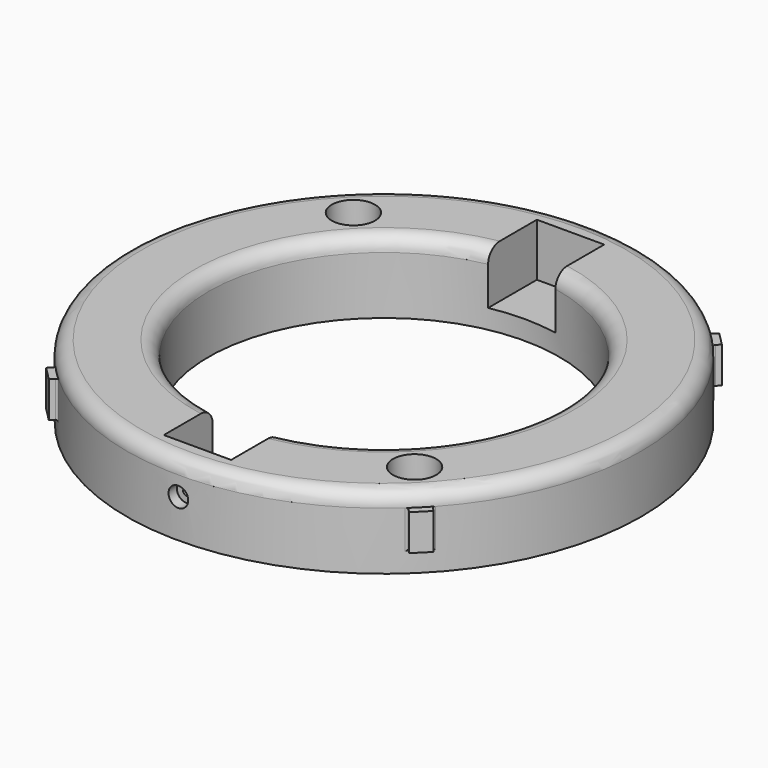
from build123d import *

# Parameters (mm, degrees)
F0_R             = 53.5
F0_R_2           = 36.5
F1_DEPTH         = 15
F5_D             = 6
F5_CBORE_D       = 9
F5_CBORE_DEPTH   = 5
F7_W             = 14
F7_H             = 11
F8_DEPTH         = 15
F10_W            = 14
F10_H            = 11
F11_DEPTH        = 15
F13_R            = 2.05
F14_DEPTH        = 2.2
F16_R            = 2.05
F17_DEPTH        = 2.2
F18_R            = 3
F19_DEPTH        = 7.5
F20_DEPTH        = 7.5
F21_R            = 3
F22_R            = 3
F25_W            = 4
F25_H            = 7.5
F26_DEPTH        = 1.5
F26_COPIES_COUNT = 4
F27_R            = 0.5
F29_D            = 1.5


# Not quite as in the source:
# - a pattern or mirror of a feature is missing from the dataset's text; its kind, count and spacing are read off the source's solid


with BuildPart() as f1:
    # F0 (on Top) → F1 (new body)
    with BuildSketch(Plane.XY):
        Circle(F0_R)
        Circle(F0_R_2, mode=Mode.SUBTRACT)
    extrude(amount=F1_DEPTH)

    # F5 (through all)
    with Locations(Plane.XY.offset(15)):
        with Locations((-31.8198051534, 31.8198051534), (31.8198051534, -31.8198051534)):
            CounterBoreHole(F5_D / 2, F5_CBORE_D / 2, F5_CBORE_DEPTH)

    # F7 (on plane+point) → F8 (cut)
    with BuildSketch(Plane.XZ.offset(-33.5)):
        with Locations((0, 9.5)):
            Rectangle(F7_W, F7_H)
    extrude(amount=-F8_DEPTH, mode=Mode.SUBTRACT)

    # F10 (on plane+point) → F11 (cut)
    with BuildSketch(Plane.XZ.offset(33.5)):
        with Locations((0, 9.5)):
            Rectangle(F10_W, F10_H)
    extrude(amount=F11_DEPTH, mode=Mode.SUBTRACT)

    # F13 (on plane+point) → F14 (cut)
    with BuildSketch(Plane.XZ.offset(53.5)):
        with Locations((0, 8)):
            Circle(F13_R)
    extrude(amount=-F14_DEPTH, mode=Mode.SUBTRACT)

    # F16 (on plane+point) → F17 (cut)
    with BuildSketch(Plane.XZ.offset(-53.5)):
        with Locations((0, 8)):
            Circle(F16_R)
    extrude(amount=F17_DEPTH, mode=Mode.SUBTRACT)

    # F18 (on face) → F19 (cut)
    with BuildSketch(Plane(origin=(0, 0, 0), x_dir=(1, 0, 0), z_dir=(0, 0, -1))):
        Polygon((-33.2340187158, -24.0416305603), (-39.5979797464, -30.405591591), (-30.405591591, -39.5979797464), (-24.0416305603, -33.2340187158), align=None)
        with Locations((-31.8198051534, -31.8198051534)):
            Circle(F18_R, mode=Mode.SUBTRACT)
    extrude(amount=-F19_DEPTH, mode=Mode.SUBTRACT)

    # F18 (on face) → F20 (cut)
    with BuildSketch(Plane(origin=(0, 0, 0), x_dir=(1, 0, 0), z_dir=(0, 0, -1))):
        Polygon((-33.2340187158, -24.0416305603), (-39.5979797464, -30.405591591), (-30.405591591, -39.5979797464), (-24.0416305603, -33.2340187158), align=None)
        Polygon((30.405591591, 39.5979797464), (24.0416305603, 33.2340187158), (33.2340187158, 24.0416305603), (39.5979797464, 30.405591591), align=None)
    extrude(amount=-F20_DEPTH, mode=Mode.SUBTRACT)

    # F21
    f21_edges = [f1.edges().sort_by_distance(p)[0] for p in [
        (-36.5, 0, 15),
    ]]
    fillet(f21_edges, radius=F21_R)

    # F22
    f22_edges = [f1.edges().sort_by_distance(p)[0] for p in [
        (-53.5, 0, 15),
        (28.175787, 23.202909, 15),
        (28.175787, -23.202909, 15),
    ]]
    fillet(f22_edges, radius=F22_R)

    # F25 (on face) → F26 (join, symmetric)
    with BuildSketch(Plane(origin=(37.8302127935, 37.8302127935, 0), x_dir=(-0.7071067812, 0.7071067812, 0), z_dir=(0.7071067812, 0.7071067812, 0))):
        with Locations((0, 8.25)):
            Rectangle(F25_W, F25_H)
    f26 = extrude(amount=F26_DEPTH, both=True)

    # F26_copies: F26 ×4 about axis
    f26_copies_axis = Axis((0, 0, 0), (0, 0, 1))
    for i in range(1, F26_COPIES_COUNT):
        add(f26.rotate(f26_copies_axis, i * 360 / F26_COPIES_COUNT))

    # F27
    f27_edges = [f1.edges().sort_by_distance(p)[0] for p in [
        (39.217983, 36.389556, 8.25),
        (36.389556, 39.217983, 8.25),
        (37.830213, 37.830213, 4.5),
        (39.217983, -36.389556, 8.25),
        (37.830213, -37.830213, 4.5),
        (36.389556, -39.217983, 8.25),
        (-36.389556, -39.217983, 8.25),
        (-37.830213, -37.830213, 4.5),
        (-39.217983, -36.389556, 8.25),
        (-39.217983, 36.389556, 8.25),
        (-37.830213, 37.830213, 4.5),
        (-36.389556, 39.217983, 8.25),
    ]]
    fillet(f27_edges, radius=F27_R)

    # F29 (through all)
    with Locations(Plane(origin=(0, 51.3, 0), x_dir=(-1, 0, 0), z_dir=(0, 1, 0))):
        with Locations((0, 8)):
            Hole(F29_D / 2)


solid = f1.part
